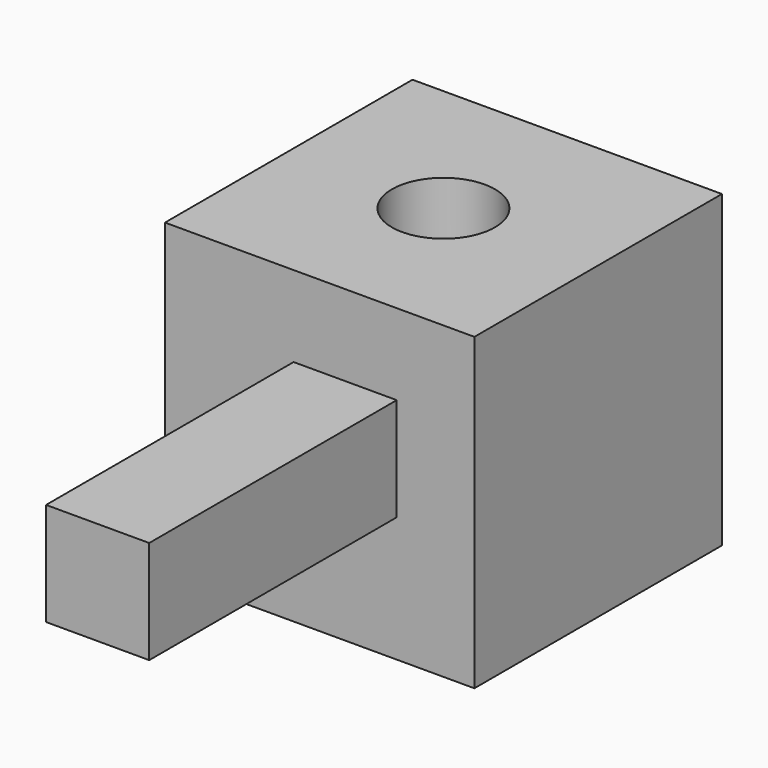
from build123d import *

# Parameters (mm, degrees)
F0_W      = 76.2
F0_H      = 76.2
F1_DEPTH  = 76.2
F3_D      = 25.4
F4_W      = 25.4
F4_H      = 25.4
F5_DEPTH  = 76.2
F10_DEPTH = 12.7
F12_DEPTH = 12.7


# Not quite as in the source:
# - the program builds the solid bodies; features that only make, move or delete a surface that nothing else refers to are left out


with BuildPart() as f1:
    # F0 (on Front) → F1 (new body)
    with BuildSketch(Plane.XZ):
        with Locations((38.1, 38.1)):
            Rectangle(F0_W, F0_H)
    extrude(amount=F1_DEPTH)

    # F3 (through all)
    with Locations(Plane.XY.offset(76.2)):
        with Locations((38.1, -38.1)):
            Hole(F3_D / 2)

    # F4 (on face) → F5 (join)
    with BuildSketch(Plane.XZ.offset(76.2)):
        with Locations((44.375465405, 43.5601483703)):
            Rectangle(F4_W, F4_H)
    extrude(amount=F5_DEPTH)

    # F9 (on face) → F10 (join)
    with BuildSketch(Plane(origin=(0, 0, 0), x_dir=(0, -1, 0), z_dir=(-1, 0, 0))):
        Polygon((52.085519187, 37.4724815469), (45.6362065152, 49.8980556745), (31.6506873282, 50.5255741276), (24.114480813, 38.7275184531), (30.5637934848, 26.3019443255), (44.5493126718, 25.6744258724), align=None)
    extrude(amount=F10_DEPTH)

    # F11 (on face) → F12 (join)
    with BuildSketch(Plane(origin=(0, 0, 0), x_dir=(-1, 0, 0), z_dir=(0, 1, 0))):
        with BuildLine():
            add(Edge.make_bspline(
                [(-48.0585680543, 49.9470105327), (-70.7842466593, 26.0252415357), (-45.6101675869, 24.8654493741), (-20.4360885145, 23.7056572126), (-22.884488982, 48.7872183711), (-25.3328894494, 73.8687795297), (-48.0585680543, 49.9470105327)],
                knots=[4.7123889804, 4.7123889804, 4.7123889804, 6.8067840828, 6.8067840828, 8.9011791852, 8.9011791852, 10.9955742876, 10.9955742876, 10.9955742876], degree=2, weights=[1, 0.5, 1, 0.5, 1, 0.5, 1]))
        make_face()
    extrude(amount=F12_DEPTH)


solid = f1.part
